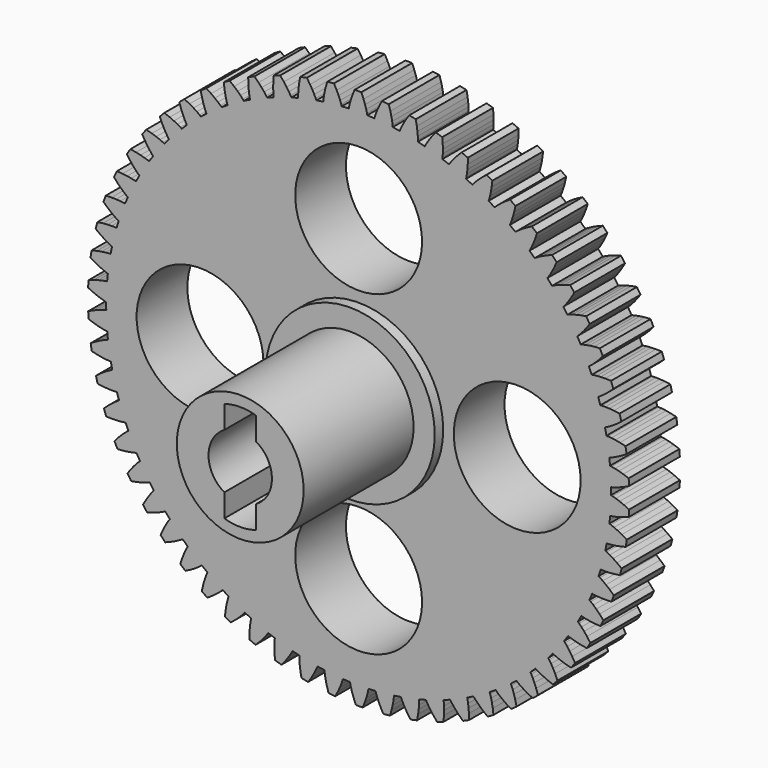
from build123d import *

# Parameters (mm, degrees)
F0_R     = 6
F0_R_2   = 3
F1_DEPTH = 20
F0_R_3   = 8
F2_DEPTH = 6
F3_DEPTH = 7
F5_DEPTH = 6
F6_R     = 6
F7_DEPTH = 6
F8_DEPTH = 10


# Not quite as in the source:
# - ends of sketch curves that miss each other by under 0.0002 mm in the source are joined


with BuildPart() as f1:
    # F0 (on Front) → F1 (new body)
    with BuildSketch(Plane.XZ):
        Circle(F0_R)
        Circle(F0_R_2, mode=Mode.SUBTRACT)
        Circle(F0_R_2)
    extrude(amount=F1_DEPTH)

    # F0 (on Front) → F2 (join)
    with BuildSketch(Plane.XZ):
        Circle(F0_R_3)
        Circle(F0_R, mode=Mode.SUBTRACT)
    extrude(amount=F2_DEPTH)

    # F0 (on Front) → F3 (join)
    with BuildSketch(Plane.XZ):
        Circle(F0_R_3)
        Circle(F0_R, mode=Mode.SUBTRACT)
    extrude(amount=F3_DEPTH)

    # F4 (on face) → F5 (cut)
    with BuildSketch(Plane.XZ.offset(20)):
        with BuildLine():
            Line((-1.5, 4.7696960071), (-1.5, 2.5980762114))
            ThreePointArc((-1.5, 2.5980762114), (-3, 0), (-1.5, -2.5980762114))
            Line((-1.5, -2.5980762114), (-1.5, -4.7696960071))
            ThreePointArc((-1.5, -4.7696960071), (0, -5), (1.5, -4.7696960071))
            Line((1.5, -4.7696960071), (1.5, -2.5980762114))
            ThreePointArc((1.5, -2.5980762114), (3, 0), (1.5, 2.5980762114))
            Line((1.5, 2.5980762114), (1.5, 4.7696960071))
            ThreePointArc((1.5, 4.7696960071), (0, 5), (-1.5, 4.7696960071))
        make_face()
    extrude(amount=-F5_DEPTH, mode=Mode.SUBTRACT)

    # F6 (on Front) → F7 (join)
    with BuildSketch(Plane.XZ):
        with BuildLine():
            Line((18.427707, 15.409639), (18.293557, 15.340559))
            ThreePointArc((18.293557, 15.340559), (18.0773970996, 15.5947006853), (17.8577068981, 15.8457969096))
            Line((17.8577068981, 15.8457969096), (17.945716, 15.968364))
            Line((17.945716, 15.968364), (18.119396, 16.237608))
            Line((18.119396, 16.237608), (18.308534, 16.565645))
            Line((18.308534, 16.565645), (18.507613, 16.954565))
            Line((18.507613, 16.954565), (18.710954, 17.406054))
            Line((18.710954, 17.406054), (18.729058, 17.452289))
            ThreePointArc((18.729058, 17.452289), (18.5121728324, 17.6821790802), (18.2924661475, 17.9093741444))
            Line((18.2924661475, 17.9093741444), (18.24545, 17.893409))
            Line((18.24545, 17.893409), (17.785115, 17.710978))
            Line((17.785115, 17.710978), (17.387477, 17.529936))
            Line((17.387477, 17.529936), (17.051116, 17.356034))
            Line((17.051116, 17.356034), (16.774193, 17.194877))
            Line((16.774193, 17.194877), (16.64772, 17.11258))
            ThreePointArc((16.64772, 17.11258), (16.4069582045, 17.3435491707), (16.1629922885, 17.5711313136))
            Line((16.1629922885, 17.5711313136), (16.238149, 17.701974))
            Line((16.238149, 17.701974), (16.3837, 17.987407))
            Line((16.3837, 17.987407), (16.53868, 18.332895))
            Line((16.53868, 18.332895), (16.697392, 18.739961))
            Line((16.697392, 18.739961), (16.854013, 19.209705))
            Line((16.854013, 19.209705), (16.867346, 19.257534))
            ThreePointArc((16.867346, 19.257534), (16.6283164042, 19.4643030587), (16.3867520575, 19.668105069))
            Line((16.3867520575, 19.668105069), (16.341592, 19.647465))
            Line((16.341592, 19.647465), (15.902075, 19.419398))
            Line((15.902075, 19.419398), (15.524793, 19.199057))
            Line((15.524793, 19.199057), (15.207751, 18.992018))
            Line((15.207751, 18.992018), (14.948553, 18.803673))
            Line((14.948553, 18.803673), (14.831055, 18.709002))
            ThreePointArc((14.831055, 18.709002), (14.5681618287, 18.9144293145), (14.302423277, 19.1161623702))
            Line((14.302423277, 19.1161623702), (14.363958, 19.253937))
            Line((14.363958, 19.253937), (14.479885, 19.552631))
            Line((14.479885, 19.552631), (14.599118, 19.912026))
            Line((14.599118, 19.912026), (14.715832, 20.333059))
            Line((14.715832, 20.333059), (14.824126, 20.816239))
            Line((14.824126, 20.816239), (14.832553, 20.865171))
            ThreePointArc((14.832553, 20.865171), (14.5738307419, 21.0466970688), (14.3128870434, 21.2250150644))
            Line((14.3128870434, 21.2250150644), (14.270048, 21.199912))
            Line((14.270048, 21.199912), (13.855859, 20.92855))
            Line((13.855859, 20.92855), (13.502804, 20.67117))
            Line((13.502804, 20.67117), (13.208334, 20.433119))
            Line((13.208334, 20.433119), (12.969521, 20.219517))
            Line((12.969521, 20.219517), (12.862204, 20.113446))
            ThreePointArc((12.862204, 20.113446), (12.5798761633, 20.2912220203), (12.2950918877, 20.4650358131))
            Line((12.2950918877, 20.4650358131), (12.342372, 20.608329))
            Line((12.342372, 20.608329), (12.427486, 20.917218))
            Line((12.427486, 20.917218), (12.509748, 21.286832))
            Line((12.509748, 21.286832), (12.583269, 21.717513))
            Line((12.583269, 21.717513), (12.642125, 22.209169))
            Line((12.642125, 22.209169), (12.645558, 22.258703))
            ThreePointArc((12.645558, 22.258703), (12.3697982504, 22.4131231925), (12.0921530789, 22.5641271472))
            Line((12.0921530789, 22.5641271472), (12.052073, 22.534819))
            Line((12.052073, 22.534819), (11.667462, 22.222946))
            Line((11.667462, 22.222946), (11.342258, 21.931169))
            Line((11.342258, 21.931169), (11.073382, 21.664548))
            Line((11.073382, 21.664548), (10.857404, 21.427882))
            Line((10.857404, 21.427882), (10.761368, 21.311498))
            ThreePointArc((10.761368, 21.311498), (10.4625040275, 21.4597992729), (10.1615969508, 21.6039098954))
            Line((10.1615969508, 21.6039098954), (10.194138, 21.751251))
            Line((10.194138, 21.751251), (10.247565, 22.067167))
            Line((10.247565, 22.067167), (10.292011, 22.443206))
            Line((10.292011, 22.443206), (10.321583, 22.879116))
            Line((10.321583, 22.879116), (10.330398, 23.374204))
            Line((10.330398, 23.374204), (10.328802, 23.423831))
            ThreePointArc((10.328802, 23.423831), (10.0388349153, 23.5495603684), (9.7473378043, 23.6717005247))
            Line((9.7473378043, 23.6717005247), (9.710428, 23.638488))
            Line((9.710428, 23.638488), (9.359342, 23.289305))
            Line((9.359342, 23.289305), (9.065325, 22.966125))
            Line((9.065325, 22.966125), (8.824802, 22.67367))
            Line((8.824802, 22.67367), (8.633875, 22.416368))
            Line((8.633875, 22.416368), (8.550107, 22.290865))
            ThreePointArc((8.550107, 22.290865), (8.2377723507, 22.4081699846), (7.9238290637, 22.5210991812))
            Line((7.9238290637, 22.5210991812), (7.941297, 22.670976))
            Line((7.941297, 22.670976), (7.96249, 22.990676))
            Line((7.96249, 22.990676), (7.968665, 23.369283))
            Line((7.968665, 23.369283), (7.953985, 23.805948))
            Line((7.953985, 23.805948), (7.912667, 24.299387))
            Line((7.912667, 24.299387), (7.906058, 24.348598))
            ThreePointArc((7.906058, 24.348598), (7.6048590633, 24.4443473758), (7.3025008735, 24.536370575))
            Line((7.3025008735, 24.536370575), (7.269141, 24.499594))
            Line((7.269141, 24.499594), (6.955183, 24.116684))
            Line((6.955183, 24.116684), (6.69537, 23.765417))
            Line((6.69537, 23.765417), (6.485668, 23.450129))
            Line((6.485668, 23.450129), (6.321751, 23.174832))
            Line((6.321751, 23.174832), (6.25111, 23.041497))
            ThreePointArc((6.25111, 23.041497), (5.9285104467, 23.1266024146), (5.6047530249, 23.207191103))
            Line((5.6047530249, 23.207191103), (5.606968, 23.358066))
            Line((5.606968, 23.358066), (5.595709, 23.67827))
            Line((5.595709, 23.67827), (5.563549, 24.055559))
            Line((5.563549, 24.055559), (5.504768, 24.488498))
            Line((5.504768, 24.488498), (5.413741, 24.975226))
            Line((5.413741, 24.975226), (5.402188, 25.023516))
            ThreePointArc((5.402188, 25.023516), (5.0928476534, 25.0883021103), (4.7827310162, 25.1492640852))
            Line((4.7827310162, 25.1492640852), (4.753263, 25.109301))
            Line((4.753263, 25.109301), (4.479653, 24.696594))
            Line((4.479653, 24.696594), (4.25671, 24.320843))
            Line((4.25671, 24.320843), (4.079982, 23.985958))
            Line((4.079982, 23.985958), (3.944758, 23.69549))
            Line((3.944758, 23.69549), (3.887967, 23.555693))
            ThreePointArc((3.887967, 23.555693), (3.5584129889, 23.6077248451), (3.2281640008, 23.6551460056))
            Line((3.2281640008, 23.6551460056), (3.215104, 23.805471))
            Line((3.215104, 23.805471), (3.171508, 24.122893))
            Line((3.171508, 24.122893), (3.101344, 24.494993))
            Line((3.101344, 24.494993), (2.999064, 24.919764))
            Line((2.999064, 24.919764), (2.859263, 25.394786))
            Line((2.859263, 25.394786), (2.842884, 25.441659))
            ThreePointArc((2.842884, 25.441659), (2.5285762096, 25.4748170229), (2.2138830225, 25.5040922591))
            Line((2.2138830225, 25.5040922591), (2.188609, 25.461353))
            Line((2.188609, 25.461353), (1.958157, 25.023082))
            Line((1.958157, 25.023082), (1.774372, 24.626705))
            Line((1.774372, 24.626705), (1.63243, 24.275659))
            Line((1.63243, 24.275659), (1.527285, 23.973001))
            Line((1.527285, 23.973001), (1.48493, 23.828176))
            ThreePointArc((1.48493, 23.828176), (1.1518024603, 23.8465998929), (0.8184500011, 23.8603670331))
            Line((0.8184500011, 23.8603670331), (0.790249, 24.0086))
            Line((0.790249, 24.0086), (0.714763, 24.319983))
            Line((0.714763, 24.319983), (0.607315, 24.683075))
            Line((0.607315, 24.683075), (0.462586, 25.095319))
            Line((0.462586, 25.095319), (0.275445, 25.55376))
            Line((0.275445, 25.55376), (0.254408, 25.598736))
            ThreePointArc((0.254408, 25.598736), (-0.0616416973, 25.599925787), (-0.3776819976, 25.5972138388))
            Line((-0.3776819976, 25.5972138388), (-0.398502, 25.552137))
            Line((-0.398502, 25.552137), (-0.583433, 25.0928))
            Line((-0.583433, 25.0928), (-0.726174, 24.679864))
            Line((-0.726174, 24.679864), (-0.831874, 24.316259))
            Line((-0.831874, 24.316259), (-0.905859, 24.004516))
            Line((-0.905859, 24.004516), (-0.933346, 23.856149))
            ThreePointArc((-0.933346, 23.856149), (-1.2666276934, 23.8407766158), (-1.5996620303, 23.8207484506))
            Line((-1.5996620303, 23.8207484506), (-1.642715, 23.965368))
            Line((-1.642715, 23.965368), (-1.749316, 24.267516))
            Line((-1.749316, 24.267516), (-1.892947, 24.617875))
            Line((-1.892947, 24.617875), (-2.078638, 25.013362))
            Line((-2.078638, 25.013362), (-2.311199, 25.450518))
            Line((-2.311199, 25.450518), (-2.336678, 25.493135))
            ThreePointArc((-2.336678, 25.493135), (-2.6512265744, 25.4623447006), (-2.9653710467, 25.4276734004))
            Line((-2.9653710467, 25.4276734004), (-2.981524, 25.380722))
            Line((-2.981524, 25.380722), (-3.119036, 24.905032))
            Line((-3.119036, 24.905032), (-3.219269, 24.479773))
            Line((-3.219269, 24.479773), (-3.287641, 24.10734))
            Line((-3.287641, 24.10734), (-3.329708, 23.789712))
            Line((-3.329708, 23.789712), (-3.342044, 23.639326))
            ThreePointArc((-3.342044, 23.639326), (-3.6720605137, 23.5903146851), (-4.0013599573, 23.5366967489))
            Line((-4.0013599573, 23.5366967489), (-4.058823, 23.676218))
            Line((-4.058823, 23.676218), (-4.195444, 23.966032))
            Line((-4.195444, 23.966032), (-4.373784, 24.300062))
            Line((-4.373784, 24.300062), (-4.598533, 24.674734))
            Line((-4.598533, 24.674734), (-4.874127, 25.08612))
            Line((-4.874127, 25.08612), (-4.903787, 25.12594))
            ThreePointArc((-4.903787, 25.12594), (-5.2136068011, 25.0634854744), (-5.5226319074, 24.9972105807))
            Line((-5.5226319074, 24.9972105807), (-5.533952, 24.948866))
            Line((-5.533952, 24.948866), (-5.622634, 24.461705))
            Line((-5.622634, 24.461705), (-5.67933, 24.028488))
            Line((-5.67933, 24.028488), (-5.709672, 23.651048))
            Line((-5.709672, 23.651048), (-5.719389, 23.330794))
            Line((-5.719389, 23.330794), (-5.716447, 23.179931))
            ThreePointArc((-5.716447, 23.179931), (-6.0398127205, 23.0977842587), (-6.3619988788, 23.0111265614))
            Line((-6.3619988788, 23.0111265614), (-6.433282, 23.144119))
            Line((-6.433282, 23.144119), (-6.598522, 23.418624))
            Line((-6.598522, 23.418624), (-6.80974, 23.732898))
            Line((-6.80974, 23.732898), (-7.071241, 24.08291))
            Line((-7.071241, 24.08291), (-7.38704, 24.464304))
            Line((-7.38704, 24.464304), (-7.420577, 24.500919))
            ThreePointArc((-7.420577, 24.500919), (-7.7224884704, 24.407440911), (-8.0232228652, 24.3102425915))
            Line((-8.0232228652, 24.3102425915), (-8.029594, 24.261))
            Line((-8.029594, 24.261), (-8.068536, 23.767367))
            Line((-8.068536, 23.767367), (-8.081113, 23.330637))
            Line((-8.081113, 23.330637), (-8.073114, 22.952065))
            Line((-8.073114, 22.952065), (-8.050382, 22.63247))
            Line((-8.050382, 22.63247), (-8.032193, 22.482679))
            ThreePointArc((-8.032193, 22.482679), (-8.3455884592, 22.3682392832), (-8.657354131, 22.2494313368))
            Line((-8.657354131, 22.2494313368), (-8.741726, 22.37453))
            Line((-8.741726, 22.37453), (-8.93389, 22.630909))
            Line((-8.93389, 22.630909), (-9.175818, 22.922202))
            Line((-9.175818, 22.922202), (-9.471389, 23.243963))
            Line((-9.471389, 23.243963), (-9.824152, 23.591451))
            Line((-9.824152, 23.591451), (-9.861221, 23.624486))
            ThreePointArc((-9.861221, 23.624486), (-10.1521265217, 23.5009431106), (-10.4414848116, 23.3738185783))
            Line((-10.4414848116, 23.3738185783), (-10.442842, 23.324184))
            Line((-10.442842, 23.324184), (-10.431643, 22.829145))
            Line((-10.431643, 22.829145), (-10.399972, 22.393382))
            Line((-10.399972, 22.393382), (-10.353716, 22.017562))
            Line((-10.353716, 22.017562), (-10.298767, 21.701907))
            Line((-10.298767, 21.701907), (-10.265517, 21.554724))
            ThreePointArc((-10.265517, 21.554724), (-10.5657271456, 21.4091659166), (-10.8638738161, 21.2594266401))
            Line((-10.8638738161, 21.2594266401), (-10.960469, 21.375348))
            Line((-10.960469, 21.375348), (-11.177584, 21.610971))
            Line((-11.177584, 21.610971), (-11.447741, 21.876294))
            Line((-11.447741, 21.876294), (-11.774347, 22.166501))
            Line((-11.774347, 22.166501), (-12.160455, 22.476518))
            Line((-12.160455, 22.476518), (-12.200676, 22.505633))
            ThreePointArc((-12.200676, 22.505633), (-12.4775902519, 22.3532937507), (-12.7526028007, 22.197547653))
            Line((-12.7526028007, 22.197547653), (-12.748931, 22.148031))
            Line((-12.748931, 22.148031), (-12.687708, 21.656664))
            Line((-12.687708, 21.656664), (-12.612114, 21.226341))
            Line((-12.612114, 21.226341), (-12.528074, 20.857129))
            Line((-12.528074, 20.857129), (-12.441473, 20.548652))
            Line((-12.441473, 20.548652), (-12.393504, 20.405589))
            ThreePointArc((-12.393504, 20.405589), (-12.6774471719, 20.2304055462), (-12.95891487, 20.0512717989))
            Line((-12.95891487, 20.0512717989), (-13.066742, 20.156825))
            Line((-13.066742, 20.156825), (-13.306581, 20.369274))
            Line((-13.306581, 20.369274), (-13.602194, 20.605905))
            Line((-13.602194, 20.605905), (-13.956484, 20.861581))
            Line((-13.956484, 20.861581), (-14.371975, 21.130945))
            Line((-14.371975, 21.130945), (-14.414935, 21.155842))
            ThreePointArc((-14.414935, 21.155842), (-14.6750168049, 20.9762694914), (-14.9328618888, 20.7934998451))
            Line((-14.9328618888, 20.7934998451), (-14.9242, 20.744608))
            Line((-14.9242, 20.744608), (-14.81358, 20.261956))
            Line((-14.81358, 20.261956), (-14.694839, 19.841489))
            Line((-14.694839, 19.841489), (-14.573877, 19.482673))
            Line((-14.573877, 19.482673), (-14.456513, 19.184541))
            Line((-14.456513, 19.184541), (-14.394316, 19.047064))
            ThreePointArc((-14.394316, 19.047064), (-14.6590798726, 18.844053509), (-14.9209810231, 18.6373630288))
            Line((-14.9209810231, 18.6373630288), (-15.038933, 18.731467))
            Line((-15.038933, 18.731467), (-15.299035, 18.918562))
            Line((-15.299035, 18.918562), (-15.617071, 19.124071))
            Line((-15.617071, 19.124071), (-15.995409, 19.342593))
            Line((-15.995409, 19.342593), (-16.43602, 19.568541))
            Line((-16.43602, 19.568541), (-16.481278, 19.588963))
            ThreePointArc((-16.481278, 19.588963), (-16.7218582, 19.3840000603), (-16.9598896372, 19.1760825898))
            Line((-16.9598896372, 19.1760825898), (-16.946326, 19.128318))
            Line((-16.946326, 19.128318), (-16.787444, 18.659334))
            Line((-16.787444, 18.659334), (-16.626775, 18.253037))
            Line((-16.626775, 18.253037), (-16.470133, 17.908299))
            Line((-16.470133, 17.908299), (-16.323209, 17.62357))
            Line((-16.323209, 17.62357), (-16.247423, 17.493091))
            ThreePointArc((-16.247423, 17.493091), (-16.4902901617, 17.2643362382), (-16.7299370859, 17.0322100874))
            Line((-16.7299370859, 17.0322100874), (-16.856804, 17.113898))
            Line((-16.856804, 17.113898), (-17.1345, 17.273719))
            Line((-17.1345, 17.273719), (-17.471695, 17.445999))
            Line((-17.471695, 17.445999), (-17.870199, 17.625124))
            Line((-17.870199, 17.625124), (-18.331408, 17.805336))
            Line((-18.331408, 17.805336), (-18.3785, 17.821075))
            ThreePointArc((-18.3785, 17.821075), (-18.5971103734, 17.5928248374), (-18.8128858824, 17.3618928915))
            Line((-18.8128858824, 17.3618928915), (-18.79456, 17.315746))
            Line((-18.79456, 17.315746), (-18.589047, 16.865241))
            Line((-18.589047, 16.865241), (-18.388097, 16.477284))
            Line((-18.388097, 16.477284), (-18.197382, 16.150162))
            Line((-18.197382, 16.150162), (-18.022407, 15.881757))
            Line((-18.022407, 15.881757), (-17.933809, 15.759615))
            ThreePointArc((-17.933809, 15.759615), (-18.1522875335, 15.5074637727), (-18.3672210142, 15.2522840118))
            Line((-18.3672210142, 15.2522840118), (-18.501702, 15.320718))
            Line((-18.501702, 15.320718), (-18.794141, 15.451625))
            Line((-18.794141, 15.451625), (-19.147036, 15.588907))
            Line((-19.147036, 15.588907), (-19.561617, 15.726797))
            Line((-19.561617, 15.726797), (-20.038692, 15.859425))
            Line((-20.038692, 15.859425), (-20.087134, 15.870319))
            ThreePointArc((-20.087134, 15.870319), (-20.2815313187, 15.6211231148), (-20.4728370145, 15.3695460109))
            Line((-20.4728370145, 15.3695460109), (-20.449936, 15.32549))
            Line((-20.449936, 15.32549), (-20.199901, 14.898088))
            Line((-20.199901, 14.898088), (-19.960733, 14.532451))
            Line((-19.960733, 14.532451), (-19.737902, 14.226302))
            Line((-19.737902, 14.226302), (-19.53667, 13.976977))
            Line((-19.53667, 13.976977), (-19.43617, 13.864424))
            ThreePointArc((-19.43617, 13.864424), (-19.6280182738, 13.5914632767), (-19.8160330616, 13.3158480414))
            Line((-19.8160330616, 13.3158480414), (-19.956747, 13.370326))
            Line((-19.956747, 13.370326), (-20.26093, 13.470975))
            Line((-20.26093, 13.470975), (-20.625902, 13.571852))
            Line((-20.625902, 13.571852), (-21.052307, 13.667092))
            Line((-21.052307, 13.667092), (-21.540351, 13.750775))
            Line((-21.540351, 13.750775), (-21.589647, 13.756712))
            ThreePointArc((-21.589647, 13.756712), (-21.757836013, 13.4891279195), (-21.92270845, 13.2194876684))
            Line((-21.92270845, 13.2194876684), (-21.895468, 13.177974))
            Line((-21.895468, 13.177974), (-21.603476, 12.778061))
            Line((-21.603476, 12.778061), (-21.328545, 12.438496))
            Line((-21.328545, 12.438496), (-21.075884, 12.156461))
            Line((-21.075884, 12.156461), (-20.850461, 11.928773))
            Line((-20.850461, 11.928773), (-20.73909, 11.826966))
            ThreePointArc((-20.73909, 11.826966), (-20.90233863, 11.5359964961), (-21.0615052823, 11.2427741507))
            Line((-21.0615052823, 11.2427741507), (-21.207009, 11.282736))
            Line((-21.207009, 11.282736), (-21.519813, 11.352096))
            Line((-21.519813, 11.352096), (-21.893119, 11.415531))
            Line((-21.893119, 11.415531), (-22.326971, 11.467144))
            Line((-22.326971, 11.467144), (-22.820977, 11.501023))
            Line((-22.820977, 11.501023), (-22.870621, 11.501942))
            ThreePointArc((-22.870621, 11.501942), (-23.0108761814, 11.2187154954), (-23.1476236456, 10.9337788326))
            Line((-23.1476236456, 10.9337788326), (-23.116323, 10.895235))
            Line((-23.116323, 10.895235), (-22.785371, 10.526914))
            Line((-22.785371, 10.526914), (-22.477497, 10.216905))
            Line((-22.477497, 10.216905), (-22.1976, 9.961878))
            Line((-22.1976, 9.961878), (-21.950298, 9.758164))
            Line((-21.950298, 9.758164), (-21.829199, 9.668146))
            ThreePointArc((-21.829199, 9.668146), (-21.9621730348, 9.3621541832), (-22.0908580775, 9.0543340318))
            Line((-22.0908580775, 9.0543340318), (-22.239658, 9.079371))
            Line((-22.239658, 9.079371), (-22.557875, 9.116729))
            Line((-22.557875, 9.116729), (-22.935682, 9.142072))
            Line((-22.935682, 9.142072), (-23.37253, 9.149528))
            Line((-23.37253, 9.149528), (-23.867429, 9.133255))
            Line((-23.867429, 9.133255), (-23.916912, 9.129147))
            ThreePointArc((-23.916912, 9.129147), (-24.0277934601, 8.8331841054), (-24.1350127325, 8.5358749054))
            Line((-24.1350127325, 8.5358749054), (-24.099973, 8.500695))
            Line((-24.099973, 8.500695), (-23.733456, 8.167746))
            Line((-23.733456, 8.167746), (-23.395799, 7.890475))
            Line((-23.395799, 7.890475), (-23.091537, 7.665073))
            Line((-23.091537, 7.665073), (-22.824895, 7.487423))
            Line((-22.824895, 7.487423), (-22.69531, 7.410119))
            ThreePointArc((-22.69531, 7.410119), (-22.7966455778, 7.0922440566), (-22.8935288599, 6.7729839585))
            Line((-22.8935288599, 6.7729839585), (-23.044098, 6.782839))
            Line((-23.044098, 6.782839), (-23.364462, 6.787811))
            Line((-23.364462, 6.787811), (-23.742895, 6.774803))
            Line((-23.742895, 6.774803), (-24.178256, 6.738025))
            Line((-24.178256, 6.738025), (-24.668969, 6.671767))
            Line((-24.668969, 6.671767), (-24.717782, 6.662675))
            ThreePointArc((-24.717782, 6.662675), (-24.7981528759, 6.3570129734), (-24.8747437834, 6.0503819473))
            Line((-24.8747437834, 6.0503819473), (-24.836325, 6.018927))
            Line((-24.836325, 6.018927), (-24.438005, 5.724766))
            Line((-24.438005, 5.724766), (-24.074029, 5.483077))
            Line((-24.074029, 5.483077), (-23.748525, 5.289614))
            Line((-23.748525, 5.289614), (-23.465278, 5.139851))
            Line((-23.465278, 5.139851), (-23.328537, 5.076054))
            ThreePointArc((-23.328537, 5.076054), (-23.3971937643, 4.7495578019), (-23.4612810018, 4.4221340003))
            Line((-23.4612810018, 4.4221340003), (-23.612075, 4.416705))
            Line((-23.612075, 4.416705), (-23.931298, 4.389242))
            Line((-23.931298, 4.389242), (-24.306473, 4.338014))
            Line((-24.306473, 4.338014), (-24.73588, 4.25738))
            Line((-24.73588, 4.25738), (-25.217372, 4.141818))
            Line((-25.217372, 4.141818), (-25.265015, 4.127834))
            ThreePointArc((-25.265015, 4.127834), (-25.314049972, 3.8156092589), (-25.3592265571, 3.5028029388))
            Line((-25.3592265571, 3.5028029388), (-25.317823, 3.475397))
            Line((-25.317823, 3.475397), (-24.891786, 3.223042))
            Line((-24.891786, 3.223042), (-24.505226, 3.019416))
            Line((-24.505226, 3.019416), (-24.16182, 2.859876))
            Line((-24.16182, 2.859876), (-23.864876, 2.739538))
            Line((-23.864876, 2.739538), (-23.722382, 2.689901))
            ThreePointArc((-23.722382, 2.689901), (-23.7576551502, 2.3581342461), (-23.7882886377, 2.0259069691))
            Line((-23.7882886377, 2.0259069691), (-23.93776, 2.005251))
            Line((-23.93776, 2.005251), (-24.252566, 1.945633))
            Line((-24.252566, 1.945633), (-24.620634, 1.856712))
            Line((-24.620634, 1.856712), (-25.03968, 1.73305))
            Line((-25.03968, 1.73305), (-25.507011, 1.569369))
            Line((-25.507011, 1.569369), (-25.552994, 1.550636))
            ThreePointArc((-25.552994, 1.550636), (-25.5701905541, 1.2350526418), (-25.5834892543, 0.9192810091))
            Line((-25.5834892543, 0.9192810091), (-25.539525, 0.896204))
            Line((-25.539525, 0.896204), (-25.090144, 0.688245))
            Line((-25.090144, 0.688245), (-24.684967, 0.524772))
            Line((-24.684967, 0.524772), (-24.327183, 0.400792))
            Line((-24.327183, 0.400792), (-24.019587, 0.311113))
            Line((-24.019587, 0.311113), (-23.872803, 0.276146))
            ThreePointArc((-23.872803, 0.276146), (-23.8743307896, -0.0574866158), (-23.8711962392, -0.3911080039))
            Line((-23.8711962392, -0.3911080039), (-24.01781, -0.426781))
            Line((-24.01781, -0.426781), (-24.32497, -0.517941))
            Line((-24.32497, -0.517941), (-24.682154, -0.643642))
            Line((-24.682154, -0.643642), (-25.086539, -0.809064))
            Line((-25.086539, -0.809064), (-25.534913, -1.019185))
            Line((-25.534913, -1.019185), (-25.578766, -1.042473))
            ThreePointArc((-25.578766, -1.042473), (-25.5639463946, -1.35817699), (-25.5452307758, -1.6736739853))
            Line((-25.5452307758, -1.6736739853), (-25.499157, -1.692185))
            Line((-25.499157, -1.692185), (-25.031044, -1.853614))
            Line((-25.031044, -1.853614), (-24.611407, -1.975257))
            Line((-24.611407, -1.975257), (-24.242915, -2.062404))
            Line((-24.242915, -2.062404), (-23.927825, -2.120505))
            Line((-23.927825, -2.120505), (-23.778257, -2.140442))
            ThreePointArc((-23.778257, -2.140442), (-23.7460235194, -2.4725174165), (-23.709153135, -2.804110016))
            Line((-23.709153135, -2.804110016), (-23.851406, -2.854433))
            Line((-23.851406, -2.854433), (-24.147768, -2.9762))
            Line((-24.147768, -2.9762), (-24.490402, -3.137392))
            Line((-24.490402, -3.137392), (-24.875976, -3.342876))
            Line((-24.875976, -3.342876), (-25.300792, -3.59728))
            Line((-25.300792, -3.59728), (-25.342064, -3.624885))
            ThreePointArc((-25.342064, -3.624885), (-25.2953815114, -3.9374705326), (-25.2448435208, -4.2494559193))
            Line((-25.2448435208, -4.2494559193), (-25.197134, -4.26321))
            Line((-25.197134, -4.26321), (-24.71509, -4.376452))
            Line((-24.71509, -4.376452), (-24.285301, -4.455017))
            Line((-24.285301, -4.455017), (-23.909883, -4.504438))
            Line((-23.909883, -4.504438), (-23.590531, -4.530363))
            Line((-23.590531, -4.530363), (-23.439713, -4.535066))
            ThreePointArc((-23.439713, -4.535066), (-23.3740498752, -4.8621772688), (-23.3038218768, -5.1883389726))
            Line((-23.3038218768, -5.1883389726), (-23.440254, -5.252794))
            Line((-23.440254, -5.252794), (-23.722776, -5.403919))
            Line((-23.722776, -5.403919), (-24.047345, -5.598948))
            Line((-24.047345, -5.598948), (-24.410153, -5.842386))
            Line((-24.410153, -5.842386), (-24.807051, -6.138462))
            Line((-24.807051, -6.138462), (-24.845318, -6.170101))
            ThreePointArc((-24.845318, -6.170101), (-24.767251878, -6.4763596574), (-24.6854102658, -6.781631073))
            Line((-24.6854102658, -6.781631073), (-24.636554, -6.790489))
            Line((-24.636554, -6.790489), (-24.145527, -6.854382))
            Line((-24.145527, -6.854382), (-23.709994, -6.889063))
            Line((-23.709994, -6.889063), (-23.331502, -6.900249))
            Line((-23.331502, -6.900249), (-23.011167, -6.893734))
            Line((-23.011167, -6.893734), (-22.860646, -6.883155))
            ThreePointArc((-22.860646, -6.883155), (-22.7622268979, -7.2019443215), (-22.6593622103, -7.5193270698))
            Line((-22.6593622103, -7.5193270698), (-22.788573, -7.597255))
            Line((-22.788573, -7.597255), (-23.054357, -7.776187))
            Line((-23.054357, -7.776187), (-23.357529, -8.003051))
            Line((-23.357529, -8.003051), (-23.693848, -8.281945))
            Line((-23.693848, -8.281945), (-24.058757, -8.616656))
            Line((-24.058757, -8.616656), (-24.093626, -8.652004))
            ThreePointArc((-24.093626, -8.652004), (-23.9849764406, -8.9487935022), (-23.8726708981, -9.2442189605))
            Line((-23.8726708981, -9.2442189605), (-23.823169, -9.248088))
            Line((-23.823169, -9.248088), (-23.328198, -9.261977))
            Line((-23.328198, -9.261977), (-22.891391, -9.252418))
            Line((-22.891391, -9.252418), (-22.513709, -9.225255))
            Line((-22.513709, -9.225255), (-22.195676, -9.186366))
            Line((-22.195676, -9.186366), (-22.046999, -9.160613))
            ThreePointArc((-22.046999, -9.160613), (-21.9168326403, -9.4678097982), (-21.7823865156, -9.7731577827))
            Line((-21.7823865156, -9.7731577827), (-21.903051, -9.863758))
            Line((-21.903051, -9.863758), (-22.149369, -10.06866))
            Line((-22.149369, -10.06866), (-22.428034, -10.325032))
            Line((-22.428034, -10.325032), (-22.734412, -10.63652))
            Line((-22.734412, -10.63652), (-23.063586, -11.00643))
            Line((-23.063586, -11.00643), (-23.094701, -11.045125))
            ThreePointArc((-23.094701, -11.045125), (-22.9565829094, -11.3293998571), (-22.8149658271, -11.611947912))
            Line((-22.8149658271, -11.611947912), (-22.765327, -11.610789))
            Line((-22.765327, -11.610789), (-22.271489, -11.574532))
            Line((-22.271489, -11.574532), (-21.837891, -11.52083))
            Line((-21.837891, -11.52083), (-21.464895, -11.455598))
            Line((-21.464895, -11.455598), (-21.152428, -11.384733))
            Line((-21.152428, -11.384733), (-21.007119, -11.34407))
            ThreePointArc((-21.007119, -11.34407), (-20.8465422324, -11.6365223462), (-20.6818942782, -11.9267021604))
            Line((-20.6818942782, -11.9267021604), (-20.792774, -12.029045))
            Line((-20.792774, -12.029045), (-21.017098, -12.257816))
            Line((-21.017098, -12.257816), (-21.268397, -12.541064))
            Line((-21.268397, -12.541064), (-21.54169, -12.881949))
            Line((-21.54169, -12.881949), (-21.831752, -13.283264))
            Line((-21.831752, -13.283264), (-21.858793, -13.324908))
            ThreePointArc((-21.858793, -13.324908), (-21.6926240273, -13.5937508735), (-21.5231487867, -13.8605218626))
            Line((-21.5231487867, -13.8605218626), (-21.473881, -13.854347))
            Line((-21.473881, -13.854347), (-20.986246, -13.768316))
            Line((-20.986246, -13.768316), (-20.560304, -13.671023))
            Line((-20.560304, -13.671023), (-20.195822, -13.56839))
            Line((-20.195822, -13.56839), (-19.892128, -13.466277))
            Line((-19.892128, -13.466277), (-19.751678, -13.411123))
            ThreePointArc((-19.751678, -13.411123), (-19.562337749, -13.6858290635), (-19.3691776506, -13.9578627482))
            Line((-19.3691776506, -13.9578627482), (-19.469135, -14.070898))
            Line((-19.469135, -14.070898), (-19.669163, -14.321189))
            Line((-19.669163, -14.321189), (-19.890517, -14.628408))
            Line((-19.890517, -14.628408), (-20.127921, -14.995193))
            Line((-20.127921, -14.995193), (-20.375895, -15.423794))
            Line((-20.375895, -15.423794), (-20.398584, -15.46796))
            ThreePointArc((-20.398584, -15.46796), (-20.2060689502, -15.7186124572), (-20.0104743761, -15.9668693001))
            Line((-20.0104743761, -15.9668693001), (-19.962085, -15.955742))
            Line((-19.962085, -15.955742), (-19.485655, -15.820818))
            Line((-19.485655, -15.820818), (-19.071742, -15.680933))
            Line((-19.071742, -15.680933), (-18.719513, -15.541953))
            Line((-18.719513, -15.541953), (-18.427707, -15.409639))
            Line((-18.427707, -15.409639), (-18.293557, -15.340559))
            ThreePointArc((-18.293557, -15.340559), (-18.0773970996, -15.5947006853), (-17.8577068981, -15.8457969096))
            Line((-17.8577068981, -15.8457969096), (-17.945716, -15.968364))
            Line((-17.945716, -15.968364), (-18.119396, -16.237608))
            Line((-18.119396, -16.237608), (-18.308534, -16.565645))
            Line((-18.308534, -16.565645), (-18.507613, -16.954565))
            Line((-18.507613, -16.954565), (-18.710954, -17.406054))
            Line((-18.710954, -17.406054), (-18.729058, -17.452289))
            ThreePointArc((-18.729058, -17.452289), (-18.5121728324, -17.6821790802), (-18.2924661475, -17.9093741444))
            Line((-18.2924661475, -17.9093741444), (-18.24545, -17.893409))
            Line((-18.24545, -17.893409), (-17.785115, -17.710978))
            Line((-17.785115, -17.710978), (-17.387477, -17.529936))
            Line((-17.387477, -17.529936), (-17.051116, -17.356034))
            Line((-17.051116, -17.356034), (-16.774193, -17.194877))
            Line((-16.774193, -17.194877), (-16.64772, -17.11258))
            ThreePointArc((-16.64772, -17.11258), (-16.4069582045, -17.3435491707), (-16.1629922885, -17.5711313136))
            Line((-16.1629922885, -17.5711313136), (-16.238149, -17.701974))
            Line((-16.238149, -17.701974), (-16.3837, -17.987407))
            Line((-16.3837, -17.987407), (-16.53868, -18.332895))
            Line((-16.53868, -18.332895), (-16.697392, -18.739961))
            Line((-16.697392, -18.739961), (-16.854013, -19.209705))
            Line((-16.854013, -19.209705), (-16.867346, -19.257534))
            ThreePointArc((-16.867346, -19.257534), (-16.6283164042, -19.4643030587), (-16.3867520575, -19.668105069))
            Line((-16.3867520575, -19.668105069), (-16.341592, -19.647465))
            Line((-16.341592, -19.647465), (-15.902075, -19.419398))
            Line((-15.902075, -19.419398), (-15.524793, -19.199057))
            Line((-15.524793, -19.199057), (-15.207751, -18.992018))
            Line((-15.207751, -18.992018), (-14.948553, -18.803673))
            Line((-14.948553, -18.803673), (-14.831055, -18.709002))
            ThreePointArc((-14.831055, -18.709002), (-14.5681618287, -18.9144293145), (-14.302423277, -19.1161623702))
            Line((-14.302423277, -19.1161623702), (-14.363958, -19.253937))
            Line((-14.363958, -19.253937), (-14.479885, -19.552631))
            Line((-14.479885, -19.552631), (-14.599118, -19.912026))
            Line((-14.599118, -19.912026), (-14.715832, -20.333059))
            Line((-14.715832, -20.333059), (-14.824126, -20.816239))
            Line((-14.824126, -20.816239), (-14.832553, -20.865171))
            ThreePointArc((-14.832553, -20.865171), (-14.5738307419, -21.0466970688), (-14.3128870434, -21.2250150644))
            Line((-14.3128870434, -21.2250150644), (-14.270048, -21.199912))
            Line((-14.270048, -21.199912), (-13.855859, -20.92855))
            Line((-13.855859, -20.92855), (-13.502804, -20.67117))
            Line((-13.502804, -20.67117), (-13.208334, -20.433119))
            Line((-13.208334, -20.433119), (-12.969521, -20.219517))
            Line((-12.969521, -20.219517), (-12.862204, -20.113446))
            ThreePointArc((-12.862204, -20.113446), (-12.5798761633, -20.2912220203), (-12.2950918877, -20.4650358131))
            Line((-12.2950918877, -20.4650358131), (-12.342372, -20.608329))
            Line((-12.342372, -20.608329), (-12.427486, -20.917218))
            Line((-12.427486, -20.917218), (-12.509748, -21.286832))
            Line((-12.509748, -21.286832), (-12.583269, -21.717513))
            Line((-12.583269, -21.717513), (-12.642125, -22.209169))
            Line((-12.642125, -22.209169), (-12.645558, -22.258703))
            ThreePointArc((-12.645558, -22.258703), (-12.3697982504, -22.4131231925), (-12.0921530789, -22.5641271472))
            Line((-12.0921530789, -22.5641271472), (-12.052073, -22.534819))
            Line((-12.052073, -22.534819), (-11.667462, -22.222946))
            Line((-11.667462, -22.222946), (-11.342258, -21.931169))
            Line((-11.342258, -21.931169), (-11.073382, -21.664548))
            Line((-11.073382, -21.664548), (-10.857404, -21.427882))
            Line((-10.857404, -21.427882), (-10.761368, -21.311498))
            ThreePointArc((-10.761368, -21.311498), (-10.4625040275, -21.4597992729), (-10.1615969508, -21.6039098954))
            Line((-10.1615969508, -21.6039098954), (-10.194138, -21.751251))
            Line((-10.194138, -21.751251), (-10.247565, -22.067167))
            Line((-10.247565, -22.067167), (-10.292011, -22.443206))
            Line((-10.292011, -22.443206), (-10.321583, -22.879116))
            Line((-10.321583, -22.879116), (-10.330398, -23.374204))
            Line((-10.330398, -23.374204), (-10.328802, -23.423831))
            ThreePointArc((-10.328802, -23.423831), (-10.0388349153, -23.5495603684), (-9.7473378043, -23.6717005247))
            Line((-9.7473378043, -23.6717005247), (-9.710428, -23.638488))
            Line((-9.710428, -23.638488), (-9.359342, -23.289305))
            Line((-9.359342, -23.289305), (-9.065325, -22.966125))
            Line((-9.065325, -22.966125), (-8.824802, -22.67367))
            Line((-8.824802, -22.67367), (-8.633875, -22.416368))
            Line((-8.633875, -22.416368), (-8.550107, -22.290865))
            ThreePointArc((-8.550107, -22.290865), (-8.2377723507, -22.4081699846), (-7.9238290637, -22.5210991812))
            Line((-7.9238290637, -22.5210991812), (-7.941297, -22.670976))
            Line((-7.941297, -22.670976), (-7.96249, -22.990676))
            Line((-7.96249, -22.990676), (-7.968665, -23.369283))
            Line((-7.968665, -23.369283), (-7.953985, -23.805948))
            Line((-7.953985, -23.805948), (-7.912667, -24.299387))
            Line((-7.912667, -24.299387), (-7.906058, -24.348598))
            ThreePointArc((-7.906058, -24.348598), (-7.6048590633, -24.4443473758), (-7.3025008735, -24.536370575))
            Line((-7.3025008735, -24.536370575), (-7.269141, -24.499594))
            Line((-7.269141, -24.499594), (-6.955183, -24.116684))
            Line((-6.955183, -24.116684), (-6.69537, -23.765417))
            Line((-6.69537, -23.765417), (-6.485668, -23.450129))
            Line((-6.485668, -23.450129), (-6.321751, -23.174832))
            Line((-6.321751, -23.174832), (-6.25111, -23.041497))
            ThreePointArc((-6.25111, -23.041497), (-5.9285104467, -23.1266024146), (-5.6047530249, -23.207191103))
            Line((-5.6047530249, -23.207191103), (-5.606968, -23.358066))
            Line((-5.606968, -23.358066), (-5.595709, -23.67827))
            Line((-5.595709, -23.67827), (-5.563549, -24.055559))
            Line((-5.563549, -24.055559), (-5.504768, -24.488498))
            Line((-5.504768, -24.488498), (-5.413741, -24.975226))
            Line((-5.413741, -24.975226), (-5.402188, -25.023516))
            ThreePointArc((-5.402188, -25.023516), (-5.0928476534, -25.0883021103), (-4.7827310162, -25.1492640852))
            Line((-4.7827310162, -25.1492640852), (-4.753263, -25.109301))
            Line((-4.753263, -25.109301), (-4.479653, -24.696594))
            Line((-4.479653, -24.696594), (-4.25671, -24.320843))
            Line((-4.25671, -24.320843), (-4.079982, -23.985958))
            Line((-4.079982, -23.985958), (-3.944758, -23.69549))
            Line((-3.944758, -23.69549), (-3.887967, -23.555693))
            ThreePointArc((-3.887967, -23.555693), (-3.5584129889, -23.6077248451), (-3.2281640008, -23.6551460056))
            Line((-3.2281640008, -23.6551460056), (-3.215104, -23.805471))
            Line((-3.215104, -23.805471), (-3.171508, -24.122893))
            Line((-3.171508, -24.122893), (-3.101344, -24.494993))
            Line((-3.101344, -24.494993), (-2.999064, -24.919764))
            Line((-2.999064, -24.919764), (-2.859263, -25.394786))
            Line((-2.859263, -25.394786), (-2.842884, -25.441659))
            ThreePointArc((-2.842884, -25.441659), (-2.5285762096, -25.4748170229), (-2.2138830225, -25.5040922591))
            Line((-2.2138830225, -25.5040922591), (-2.188609, -25.461353))
            Line((-2.188609, -25.461353), (-1.958157, -25.023082))
            Line((-1.958157, -25.023082), (-1.774372, -24.626705))
            Line((-1.774372, -24.626705), (-1.63243, -24.275659))
            Line((-1.63243, -24.275659), (-1.527285, -23.973001))
            Line((-1.527285, -23.973001), (-1.48493, -23.828176))
            ThreePointArc((-1.48493, -23.828176), (-1.1518024603, -23.8465998929), (-0.8184500011, -23.8603670331))
            Line((-0.8184500011, -23.8603670331), (-0.790249, -24.0086))
            Line((-0.790249, -24.0086), (-0.714763, -24.319983))
            Line((-0.714763, -24.319983), (-0.607315, -24.683075))
            Line((-0.607315, -24.683075), (-0.462586, -25.095319))
            Line((-0.462586, -25.095319), (-0.275445, -25.55376))
            Line((-0.275445, -25.55376), (-0.254408, -25.598736))
            ThreePointArc((-0.254408, -25.598736), (0.0616416973, -25.599925787), (0.3776819976, -25.5972138388))
            Line((0.3776819976, -25.5972138388), (0.398502, -25.552137))
            Line((0.398502, -25.552137), (0.583433, -25.0928))
            Line((0.583433, -25.0928), (0.726174, -24.679864))
            Line((0.726174, -24.679864), (0.831874, -24.316259))
            Line((0.831874, -24.316259), (0.905859, -24.004516))
            Line((0.905859, -24.004516), (0.933346, -23.856149))
            ThreePointArc((0.933346, -23.856149), (1.2666276934, -23.8407766158), (1.5996620303, -23.8207484506))
            Line((1.5996620303, -23.8207484506), (1.642715, -23.965368))
            Line((1.642715, -23.965368), (1.749316, -24.267516))
            Line((1.749316, -24.267516), (1.892947, -24.617875))
            Line((1.892947, -24.617875), (2.078638, -25.013362))
            Line((2.078638, -25.013362), (2.311199, -25.450518))
            Line((2.311199, -25.450518), (2.336678, -25.493135))
            ThreePointArc((2.336678, -25.493135), (2.6512265744, -25.4623447006), (2.9653710467, -25.4276734004))
            Line((2.9653710467, -25.4276734004), (2.981524, -25.380722))
            Line((2.981524, -25.380722), (3.119036, -24.905032))
            Line((3.119036, -24.905032), (3.219269, -24.479773))
            Line((3.219269, -24.479773), (3.287641, -24.10734))
            Line((3.287641, -24.10734), (3.329708, -23.789712))
            Line((3.329708, -23.789712), (3.342044, -23.639326))
            ThreePointArc((3.342044, -23.639326), (3.6720605137, -23.5903146851), (4.0013599573, -23.5366967489))
            Line((4.0013599573, -23.5366967489), (4.058823, -23.676218))
            Line((4.058823, -23.676218), (4.195444, -23.966032))
            Line((4.195444, -23.966032), (4.373784, -24.300062))
            Line((4.373784, -24.300062), (4.598533, -24.674734))
            Line((4.598533, -24.674734), (4.874127, -25.08612))
            Line((4.874127, -25.08612), (4.903787, -25.12594))
            ThreePointArc((4.903787, -25.12594), (5.2136068011, -25.0634854744), (5.5226319074, -24.9972105807))
            Line((5.5226319074, -24.9972105807), (5.533952, -24.948866))
            Line((5.533952, -24.948866), (5.622634, -24.461705))
            Line((5.622634, -24.461705), (5.67933, -24.028488))
            Line((5.67933, -24.028488), (5.709672, -23.651048))
            Line((5.709672, -23.651048), (5.719389, -23.330794))
            Line((5.719389, -23.330794), (5.716447, -23.179931))
            ThreePointArc((5.716447, -23.179931), (6.0398127205, -23.0977842587), (6.3619988788, -23.0111265614))
            Line((6.3619988788, -23.0111265614), (6.433282, -23.144119))
            Line((6.433282, -23.144119), (6.598522, -23.418624))
            Line((6.598522, -23.418624), (6.80974, -23.732898))
            Line((6.80974, -23.732898), (7.071241, -24.08291))
            Line((7.071241, -24.08291), (7.38704, -24.464304))
            Line((7.38704, -24.464304), (7.420577, -24.500919))
            ThreePointArc((7.420577, -24.500919), (7.7224884704, -24.407440911), (8.0232228652, -24.3102425915))
            Line((8.0232228652, -24.3102425915), (8.029594, -24.261))
            Line((8.029594, -24.261), (8.068536, -23.767367))
            Line((8.068536, -23.767367), (8.081113, -23.330637))
            Line((8.081113, -23.330637), (8.073114, -22.952065))
            Line((8.073114, -22.952065), (8.050382, -22.63247))
            Line((8.050382, -22.63247), (8.032193, -22.482679))
            ThreePointArc((8.032193, -22.482679), (8.3455884592, -22.3682392832), (8.657354131, -22.2494313368))
            Line((8.657354131, -22.2494313368), (8.741726, -22.37453))
            Line((8.741726, -22.37453), (8.93389, -22.630909))
            Line((8.93389, -22.630909), (9.175818, -22.922202))
            Line((9.175818, -22.922202), (9.471389, -23.243963))
            Line((9.471389, -23.243963), (9.824152, -23.591451))
            Line((9.824152, -23.591451), (9.861221, -23.624486))
            ThreePointArc((9.861221, -23.624486), (10.1521265217, -23.5009431106), (10.4414848116, -23.3738185783))
            Line((10.4414848116, -23.3738185783), (10.442842, -23.324184))
            Line((10.442842, -23.324184), (10.431643, -22.829145))
            Line((10.431643, -22.829145), (10.399972, -22.393382))
            Line((10.399972, -22.393382), (10.353716, -22.017562))
            Line((10.353716, -22.017562), (10.298767, -21.701907))
            Line((10.298767, -21.701907), (10.265517, -21.554724))
            ThreePointArc((10.265517, -21.554724), (10.5657271456, -21.4091659166), (10.8638738161, -21.2594266401))
            Line((10.8638738161, -21.2594266401), (10.960469, -21.375348))
            Line((10.960469, -21.375348), (11.177584, -21.610971))
            Line((11.177584, -21.610971), (11.447741, -21.876294))
            Line((11.447741, -21.876294), (11.774347, -22.166501))
            Line((11.774347, -22.166501), (12.160455, -22.476518))
            Line((12.160455, -22.476518), (12.200676, -22.505633))
            ThreePointArc((12.200676, -22.505633), (12.4775902519, -22.3532937507), (12.7526028007, -22.197547653))
            Line((12.7526028007, -22.197547653), (12.748931, -22.148031))
            Line((12.748931, -22.148031), (12.687708, -21.656664))
            Line((12.687708, -21.656664), (12.612114, -21.226341))
            Line((12.612114, -21.226341), (12.528074, -20.857129))
            Line((12.528074, -20.857129), (12.441473, -20.548652))
            Line((12.441473, -20.548652), (12.393504, -20.405589))
            ThreePointArc((12.393504, -20.405589), (12.6774471719, -20.2304055462), (12.95891487, -20.0512717989))
            Line((12.95891487, -20.0512717989), (13.066742, -20.156825))
            Line((13.066742, -20.156825), (13.306581, -20.369274))
            Line((13.306581, -20.369274), (13.602194, -20.605905))
            Line((13.602194, -20.605905), (13.956484, -20.861581))
            Line((13.956484, -20.861581), (14.371975, -21.130945))
            Line((14.371975, -21.130945), (14.414935, -21.155842))
            ThreePointArc((14.414935, -21.155842), (14.6750168049, -20.9762694914), (14.9328618888, -20.7934998451))
            Line((14.9328618888, -20.7934998451), (14.9242, -20.744608))
            Line((14.9242, -20.744608), (14.81358, -20.261956))
            Line((14.81358, -20.261956), (14.694839, -19.841489))
            Line((14.694839, -19.841489), (14.573877, -19.482673))
            Line((14.573877, -19.482673), (14.456513, -19.184541))
            Line((14.456513, -19.184541), (14.394316, -19.047064))
            ThreePointArc((14.394316, -19.047064), (14.6590798726, -18.844053509), (14.9209810231, -18.6373630288))
            Line((14.9209810231, -18.6373630288), (15.038933, -18.731467))
            Line((15.038933, -18.731467), (15.299035, -18.918562))
            Line((15.299035, -18.918562), (15.617071, -19.124071))
            Line((15.617071, -19.124071), (15.995409, -19.342593))
            Line((15.995409, -19.342593), (16.43602, -19.568541))
            Line((16.43602, -19.568541), (16.481278, -19.588963))
            ThreePointArc((16.481278, -19.588963), (16.7218582, -19.3840000603), (16.9598896372, -19.1760825898))
            Line((16.9598896372, -19.1760825898), (16.946326, -19.128318))
            Line((16.946326, -19.128318), (16.787444, -18.659334))
            Line((16.787444, -18.659334), (16.626775, -18.253037))
            Line((16.626775, -18.253037), (16.470133, -17.908299))
            Line((16.470133, -17.908299), (16.323209, -17.62357))
            Line((16.323209, -17.62357), (16.247423, -17.493091))
            ThreePointArc((16.247423, -17.493091), (16.4902901617, -17.2643362382), (16.7299370859, -17.0322100874))
            Line((16.7299370859, -17.0322100874), (16.856804, -17.113898))
            Line((16.856804, -17.113898), (17.1345, -17.273719))
            Line((17.1345, -17.273719), (17.471695, -17.445999))
            Line((17.471695, -17.445999), (17.870199, -17.625124))
            Line((17.870199, -17.625124), (18.331408, -17.805336))
            Line((18.331408, -17.805336), (18.3785, -17.821075))
            ThreePointArc((18.3785, -17.821075), (18.5971103734, -17.5928248374), (18.8128858824, -17.3618928915))
            Line((18.8128858824, -17.3618928915), (18.79456, -17.315746))
            Line((18.79456, -17.315746), (18.589047, -16.865241))
            Line((18.589047, -16.865241), (18.388097, -16.477284))
            Line((18.388097, -16.477284), (18.197382, -16.150162))
            Line((18.197382, -16.150162), (18.022407, -15.881757))
            Line((18.022407, -15.881757), (17.933809, -15.759615))
            ThreePointArc((17.933809, -15.759615), (18.1522875335, -15.5074637727), (18.3672210142, -15.2522840118))
            Line((18.3672210142, -15.2522840118), (18.501702, -15.320718))
            Line((18.501702, -15.320718), (18.794141, -15.451625))
            Line((18.794141, -15.451625), (19.147036, -15.588907))
            Line((19.147036, -15.588907), (19.561617, -15.726797))
            Line((19.561617, -15.726797), (20.038692, -15.859425))
            Line((20.038692, -15.859425), (20.087134, -15.870319))
            ThreePointArc((20.087134, -15.870319), (20.2815313187, -15.6211231148), (20.4728370145, -15.3695460109))
            Line((20.4728370145, -15.3695460109), (20.449936, -15.32549))
            Line((20.449936, -15.32549), (20.199901, -14.898088))
            Line((20.199901, -14.898088), (19.960733, -14.532451))
            Line((19.960733, -14.532451), (19.737902, -14.226302))
            Line((19.737902, -14.226302), (19.53667, -13.976977))
            Line((19.53667, -13.976977), (19.43617, -13.864424))
            ThreePointArc((19.43617, -13.864424), (19.6280182738, -13.5914632767), (19.8160330616, -13.3158480414))
            Line((19.8160330616, -13.3158480414), (19.956747, -13.370326))
            Line((19.956747, -13.370326), (20.26093, -13.470975))
            Line((20.26093, -13.470975), (20.625902, -13.571852))
            Line((20.625902, -13.571852), (21.052307, -13.667092))
            Line((21.052307, -13.667092), (21.540351, -13.750775))
            Line((21.540351, -13.750775), (21.589647, -13.756712))
            ThreePointArc((21.589647, -13.756712), (21.757836013, -13.4891279195), (21.92270845, -13.2194876684))
            Line((21.92270845, -13.2194876684), (21.895468, -13.177974))
            Line((21.895468, -13.177974), (21.603476, -12.778061))
            Line((21.603476, -12.778061), (21.328545, -12.438496))
            Line((21.328545, -12.438496), (21.075884, -12.156461))
            Line((21.075884, -12.156461), (20.850461, -11.928773))
            Line((20.850461, -11.928773), (20.73909, -11.826966))
            ThreePointArc((20.73909, -11.826966), (20.90233863, -11.5359964961), (21.0615052823, -11.2427741507))
            Line((21.0615052823, -11.2427741507), (21.207009, -11.282736))
            Line((21.207009, -11.282736), (21.519813, -11.352096))
            Line((21.519813, -11.352096), (21.893119, -11.415531))
            Line((21.893119, -11.415531), (22.326971, -11.467144))
            Line((22.326971, -11.467144), (22.820977, -11.501023))
            Line((22.820977, -11.501023), (22.870621, -11.501942))
            ThreePointArc((22.870621, -11.501942), (23.0108761814, -11.2187154954), (23.1476236456, -10.9337788326))
            Line((23.1476236456, -10.9337788326), (23.116323, -10.895235))
            Line((23.116323, -10.895235), (22.785371, -10.526914))
            Line((22.785371, -10.526914), (22.477497, -10.216905))
            Line((22.477497, -10.216905), (22.1976, -9.961878))
            Line((22.1976, -9.961878), (21.950298, -9.758164))
            Line((21.950298, -9.758164), (21.829199, -9.668146))
            ThreePointArc((21.829199, -9.668146), (21.9621730348, -9.3621541832), (22.0908580775, -9.0543340318))
            Line((22.0908580775, -9.0543340318), (22.239658, -9.079371))
            Line((22.239658, -9.079371), (22.557875, -9.116729))
            Line((22.557875, -9.116729), (22.935682, -9.142072))
            Line((22.935682, -9.142072), (23.37253, -9.149528))
            Line((23.37253, -9.149528), (23.867429, -9.133255))
            Line((23.867429, -9.133255), (23.916912, -9.129147))
            ThreePointArc((23.916912, -9.129147), (24.0277934601, -8.8331841054), (24.1350127325, -8.5358749054))
            Line((24.1350127325, -8.5358749054), (24.099973, -8.500695))
            Line((24.099973, -8.500695), (23.733456, -8.167746))
            Line((23.733456, -8.167746), (23.395799, -7.890475))
            Line((23.395799, -7.890475), (23.091537, -7.665073))
            Line((23.091537, -7.665073), (22.824895, -7.487423))
            Line((22.824895, -7.487423), (22.69531, -7.410119))
            ThreePointArc((22.69531, -7.410119), (22.7966455778, -7.0922440566), (22.8935288599, -6.7729839585))
            Line((22.8935288599, -6.7729839585), (23.044098, -6.782839))
            Line((23.044098, -6.782839), (23.364462, -6.787811))
            Line((23.364462, -6.787811), (23.742895, -6.774803))
            Line((23.742895, -6.774803), (24.178256, -6.738025))
            Line((24.178256, -6.738025), (24.668969, -6.671767))
            Line((24.668969, -6.671767), (24.717782, -6.662675))
            ThreePointArc((24.717782, -6.662675), (24.7981528759, -6.3570129734), (24.8747437834, -6.0503819473))
            Line((24.8747437834, -6.0503819473), (24.836325, -6.018927))
            Line((24.836325, -6.018927), (24.438005, -5.724766))
            Line((24.438005, -5.724766), (24.074029, -5.483077))
            Line((24.074029, -5.483077), (23.748525, -5.289614))
            Line((23.748525, -5.289614), (23.465278, -5.139851))
            Line((23.465278, -5.139851), (23.328537, -5.076054))
            ThreePointArc((23.328537, -5.076054), (23.3971937643, -4.7495578019), (23.4612810018, -4.4221340003))
            Line((23.4612810018, -4.4221340003), (23.612075, -4.416705))
            Line((23.612075, -4.416705), (23.931298, -4.389242))
            Line((23.931298, -4.389242), (24.306473, -4.338014))
            Line((24.306473, -4.338014), (24.73588, -4.25738))
            Line((24.73588, -4.25738), (25.217372, -4.141818))
            Line((25.217372, -4.141818), (25.265015, -4.127834))
            ThreePointArc((25.265015, -4.127834), (25.314049972, -3.8156092589), (25.3592265571, -3.5028029388))
            Line((25.3592265571, -3.5028029388), (25.317823, -3.475397))
            Line((25.317823, -3.475397), (24.891786, -3.223042))
            Line((24.891786, -3.223042), (24.505226, -3.019416))
            Line((24.505226, -3.019416), (24.16182, -2.859876))
            Line((24.16182, -2.859876), (23.864876, -2.739538))
            Line((23.864876, -2.739538), (23.722382, -2.689901))
            ThreePointArc((23.722382, -2.689901), (23.7576551502, -2.3581342461), (23.7882886377, -2.0259069691))
            Line((23.7882886377, -2.0259069691), (23.93776, -2.005251))
            Line((23.93776, -2.005251), (24.252566, -1.945633))
            Line((24.252566, -1.945633), (24.620634, -1.856712))
            Line((24.620634, -1.856712), (25.03968, -1.73305))
            Line((25.03968, -1.73305), (25.507011, -1.569369))
            Line((25.507011, -1.569369), (25.552994, -1.550636))
            ThreePointArc((25.552994, -1.550636), (25.5701905541, -1.2350526418), (25.5834892543, -0.9192810091))
            Line((25.5834892543, -0.9192810091), (25.539525, -0.896204))
            Line((25.539525, -0.896204), (25.090144, -0.688245))
            Line((25.090144, -0.688245), (24.684967, -0.524772))
            Line((24.684967, -0.524772), (24.327183, -0.400792))
            Line((24.327183, -0.400792), (24.019587, -0.311113))
            Line((24.019587, -0.311113), (23.872803, -0.276146))
            ThreePointArc((23.872803, -0.276146), (23.8743307896, 0.0574866158), (23.8711962392, 0.3911080039))
            Line((23.8711962392, 0.3911080039), (24.01781, 0.426781))
            Line((24.01781, 0.426781), (24.32497, 0.517941))
            Line((24.32497, 0.517941), (24.682154, 0.643642))
            Line((24.682154, 0.643642), (25.086539, 0.809064))
            Line((25.086539, 0.809064), (25.534913, 1.019185))
            Line((25.534913, 1.019185), (25.578766, 1.042473))
            ThreePointArc((25.578766, 1.042473), (25.5639463946, 1.35817699), (25.5452307758, 1.6736739853))
            Line((25.5452307758, 1.6736739853), (25.499157, 1.692185))
            Line((25.499157, 1.692185), (25.031044, 1.853614))
            Line((25.031044, 1.853614), (24.611407, 1.975257))
            Line((24.611407, 1.975257), (24.242915, 2.062404))
            Line((24.242915, 2.062404), (23.927825, 2.120505))
            Line((23.927825, 2.120505), (23.778257, 2.140442))
            ThreePointArc((23.778257, 2.140442), (23.7460235194, 2.4725174165), (23.709153135, 2.804110016))
            Line((23.709153135, 2.804110016), (23.851406, 2.854433))
            Line((23.851406, 2.854433), (24.147768, 2.9762))
            Line((24.147768, 2.9762), (24.490402, 3.137392))
            Line((24.490402, 3.137392), (24.875976, 3.342876))
            Line((24.875976, 3.342876), (25.300792, 3.59728))
            Line((25.300792, 3.59728), (25.342064, 3.624885))
            ThreePointArc((25.342064, 3.624885), (25.2953815114, 3.9374705326), (25.2448435208, 4.2494559193))
            Line((25.2448435208, 4.2494559193), (25.197134, 4.26321))
            Line((25.197134, 4.26321), (24.71509, 4.376452))
            Line((24.71509, 4.376452), (24.285301, 4.455017))
            Line((24.285301, 4.455017), (23.909883, 4.504438))
            Line((23.909883, 4.504438), (23.590531, 4.530363))
            Line((23.590531, 4.530363), (23.439713, 4.535066))
            ThreePointArc((23.439713, 4.535066), (23.3740498752, 4.8621772688), (23.3038218768, 5.1883389726))
            Line((23.3038218768, 5.1883389726), (23.440254, 5.252794))
            Line((23.440254, 5.252794), (23.722776, 5.403919))
            Line((23.722776, 5.403919), (24.047345, 5.598948))
            Line((24.047345, 5.598948), (24.410153, 5.842386))
            Line((24.410153, 5.842386), (24.807051, 6.138462))
            Line((24.807051, 6.138462), (24.845318, 6.170101))
            ThreePointArc((24.845318, 6.170101), (24.767251878, 6.4763596574), (24.6854102658, 6.781631073))
            Line((24.6854102658, 6.781631073), (24.636554, 6.790489))
            Line((24.636554, 6.790489), (24.145527, 6.854382))
            Line((24.145527, 6.854382), (23.709994, 6.889063))
            Line((23.709994, 6.889063), (23.331502, 6.900249))
            Line((23.331502, 6.900249), (23.011167, 6.893734))
            Line((23.011167, 6.893734), (22.860646, 6.883155))
            ThreePointArc((22.860646, 6.883155), (22.7622268979, 7.2019443215), (22.6593622103, 7.5193270698))
            Line((22.6593622103, 7.5193270698), (22.788573, 7.597255))
            Line((22.788573, 7.597255), (23.054357, 7.776187))
            Line((23.054357, 7.776187), (23.357529, 8.003051))
            Line((23.357529, 8.003051), (23.693848, 8.281945))
            Line((23.693848, 8.281945), (24.058757, 8.616656))
            Line((24.058757, 8.616656), (24.093626, 8.652004))
            ThreePointArc((24.093626, 8.652004), (23.9849764406, 8.9487935022), (23.8726708981, 9.2442189605))
            Line((23.8726708981, 9.2442189605), (23.823169, 9.248088))
            Line((23.823169, 9.248088), (23.328198, 9.261977))
            Line((23.328198, 9.261977), (22.891391, 9.252418))
            Line((22.891391, 9.252418), (22.513709, 9.225255))
            Line((22.513709, 9.225255), (22.195676, 9.186366))
            Line((22.195676, 9.186366), (22.046999, 9.160613))
            ThreePointArc((22.046999, 9.160613), (21.9168326403, 9.4678097982), (21.7823865156, 9.7731577827))
            Line((21.7823865156, 9.7731577827), (21.903051, 9.863758))
            Line((21.903051, 9.863758), (22.149369, 10.06866))
            Line((22.149369, 10.06866), (22.428034, 10.325032))
            Line((22.428034, 10.325032), (22.734412, 10.63652))
            Line((22.734412, 10.63652), (23.063586, 11.00643))
            Line((23.063586, 11.00643), (23.094701, 11.045125))
            ThreePointArc((23.094701, 11.045125), (22.9565829094, 11.3293998571), (22.8149658271, 11.611947912))
            Line((22.8149658271, 11.611947912), (22.765327, 11.610789))
            Line((22.765327, 11.610789), (22.271489, 11.574532))
            Line((22.271489, 11.574532), (21.837891, 11.52083))
            Line((21.837891, 11.52083), (21.464895, 11.455598))
            Line((21.464895, 11.455598), (21.152428, 11.384733))
            Line((21.152428, 11.384733), (21.007119, 11.34407))
            ThreePointArc((21.007119, 11.34407), (20.8465422324, 11.6365223462), (20.6818942782, 11.9267021604))
            Line((20.6818942782, 11.9267021604), (20.792774, 12.029045))
            Line((20.792774, 12.029045), (21.017098, 12.257816))
            Line((21.017098, 12.257816), (21.268397, 12.541064))
            Line((21.268397, 12.541064), (21.54169, 12.881949))
            Line((21.54169, 12.881949), (21.831752, 13.283264))
            Line((21.831752, 13.283264), (21.858793, 13.324908))
            ThreePointArc((21.858793, 13.324908), (21.6926240273, 13.5937508735), (21.5231487867, 13.8605218626))
            Line((21.5231487867, 13.8605218626), (21.473881, 13.854347))
            Line((21.473881, 13.854347), (20.986246, 13.768316))
            Line((20.986246, 13.768316), (20.560304, 13.671023))
            Line((20.560304, 13.671023), (20.195822, 13.56839))
            Line((20.195822, 13.56839), (19.892128, 13.466277))
            Line((19.892128, 13.466277), (19.751678, 13.411123))
            ThreePointArc((19.751678, 13.411123), (19.562337749, 13.6858290635), (19.3691776506, 13.9578627482))
            Line((19.3691776506, 13.9578627482), (19.469135, 14.070898))
            Line((19.469135, 14.070898), (19.669163, 14.321189))
            Line((19.669163, 14.321189), (19.890517, 14.628408))
            Line((19.890517, 14.628408), (20.127921, 14.995193))
            Line((20.127921, 14.995193), (20.375895, 15.423794))
            Line((20.375895, 15.423794), (20.398584, 15.46796))
            ThreePointArc((20.398584, 15.46796), (20.2060689502, 15.7186124572), (20.0104743761, 15.9668693001))
            Line((20.0104743761, 15.9668693001), (19.962085, 15.955742))
            Line((19.962085, 15.955742), (19.485655, 15.820818))
            Line((19.485655, 15.820818), (19.071742, 15.680933))
            Line((19.071742, 15.680933), (18.719513, 15.541953))
            Line((18.719513, 15.541953), (18.427707, 15.409639))
        make_face()
        with Locations((0, -15)):
            Circle(F6_R, mode=Mode.SUBTRACT)
        with Locations((-15, 0)):
            Circle(F6_R, mode=Mode.SUBTRACT)
        with Locations((15, 0)):
            Circle(F6_R, mode=Mode.SUBTRACT)
        with Locations((0, 15)):
            Circle(F6_R, mode=Mode.SUBTRACT)
    extrude(amount=F7_DEPTH)

    # F0 (on Front) → F8 (cut)
    with BuildSketch(Plane.XZ):
        Circle(F0_R_2)
    extrude(amount=F8_DEPTH, mode=Mode.SUBTRACT)


solid = f1.part
